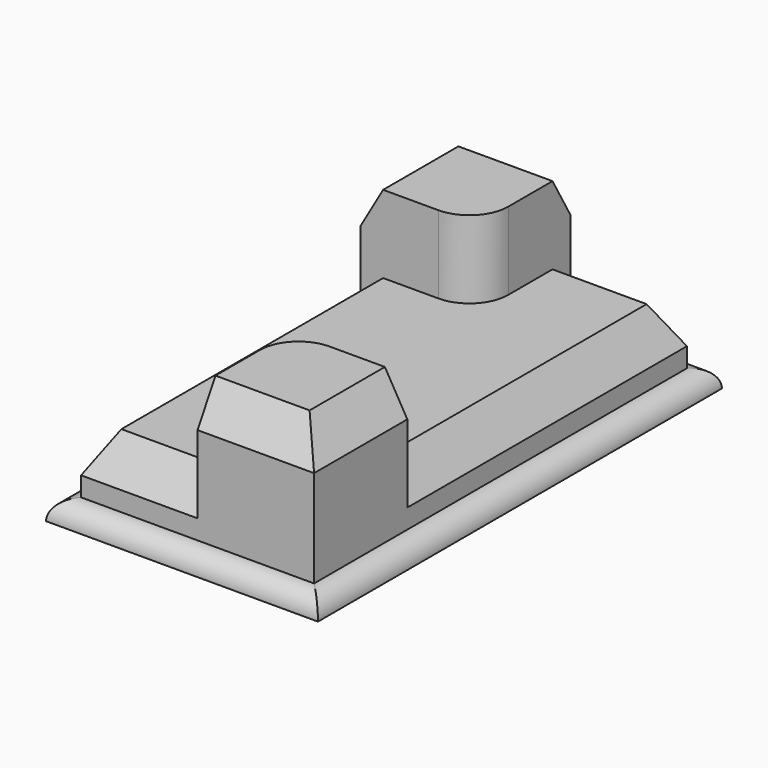
from build123d import *

# Parameters (mm, degrees)
F0_W     = 88.9
F0_H     = 165.1
F1_DEPTH = 6.35
F2_DEPTH = 25.4
F3_DEPTH = 50.8
F4_R     = 6.34999
F5_SIZE2 = 12.7
F5_SIZE  = 7.3323484187
F6_SIZE2 = 12.7
F6_SIZE  = 7.3323484187
F7_SIZE2 = 12.7
F7_SIZE  = 7.3323484187


# Not quite as in the source:
# - a fillet or chamfer is up to 0.001 mm smaller than in the source, because OpenCascade refuses the exact size


with BuildPart() as f1:
    # F0 (on Top) → F1 (new body)
    with BuildSketch(Plane.XY):
        Rectangle(F0_W, F0_H)
        Polygon((0, 76.2), (38.1, 76.2), (38.1, -38.1), (38.1, -76.2), (0, -76.2), (-38.1, -76.2), (-38.1, 38.1), (-38.1, 76.2), align=None, mode=Mode.SUBTRACT)
    extrude(amount=F1_DEPTH)

    # F0 (on Top) → F2 (join)
    with BuildSketch(Plane.XY):
        with BuildLine():
            Line((38.1, -38.1), (38.1, 76.2))
            Line((38.1, 76.2), (0, 76.2))
            Line((0, 76.2), (0, 50.8))
            ThreePointArc((0, 50.8), (-3.7197438789, 41.8197438789), (-12.7, 38.1))
            Line((-12.7, 38.1), (-38.1, 38.1))
            Line((-38.1, 38.1), (-38.1, -76.2))
            Line((-38.1, -76.2), (0, -76.2))
            Line((0, -76.2), (0, -50.8))
            ThreePointArc((0, -50.8), (3.7197438789, -41.8197438789), (12.7, -38.1))
            Line((12.7, -38.1), (38.1, -38.1))
        make_face()
    extrude(amount=F2_DEPTH)

    # F0 (on Top) → F3 (join)
    with BuildSketch(Plane.XY):
        with BuildLine():
            Line((38.1, -76.2), (38.1, -38.1))
            Line((38.1, -38.1), (12.7, -38.1))
            ThreePointArc((12.7, -38.1), (3.7197438789, -41.8197438789), (0, -50.8))
            Line((0, -50.8), (0, -76.2))
            Line((0, -76.2), (38.1, -76.2))
        make_face()
        with BuildLine():
            Line((0, 50.8), (0, 76.2))
            Line((0, 76.2), (-38.1, 76.2))
            Line((-38.1, 76.2), (-38.1, 38.1))
            Line((-38.1, 38.1), (-12.7, 38.1))
            ThreePointArc((-12.7, 38.1), (-3.7197438789, 41.8197438789), (0, 50.8))
        make_face()
    extrude(amount=F3_DEPTH)

    # F4 (radius 6.35 in the source; OpenCascade refuses exactly that, so slightly less here)
    f4_edges = [f1.edges().sort_by_distance(p)[0] for p in [
        (0, -82.55, 6.35),
        (44.45, 0, 6.35),
        (-44.45, 0, 6.35),
        (0, 82.55, 6.35),
    ]]
    fillet(f4_edges, radius=F4_R)

    # F5
    f5_edges = [f1.edges().sort_by_distance(p)[0] for p in [
        (38.1, 19.05, 25.4),
        (19.05, 76.2, 25.4),
        (-38.1, -19.05, 25.4),
        (-19.05, -76.2, 25.4),
    ]]
    f5_side = f1.faces().sort_by_distance((0, 0, 25.4))[0]
    chamfer(f5_edges, length=F5_SIZE, length2=F5_SIZE2, reference=f5_side)

    # F6
    f6_edges = [f1.edges().sort_by_distance(p)[0] for p in [
        (38.1, -57.15, 50.8),
        (19.05, -76.2, 50.8),
    ]]
    f6_side = f1.faces().sort_by_distance((19.446042, -57.546042, 50.8))[0]
    chamfer(f6_edges, length=F6_SIZE, length2=F6_SIZE2, reference=f6_side)

    # F7
    f7_edges = [f1.edges().sort_by_distance(p)[0] for p in [
        (-19.05, 76.2, 50.8),
        (-38.1, 57.15, 50.8),
    ]]
    f7_side = f1.faces().sort_by_distance((-19.446042, 57.546042, 50.8))[0]
    chamfer(f7_edges, length=F7_SIZE, length2=F7_SIZE2, reference=f7_side)


solid = f1.part
